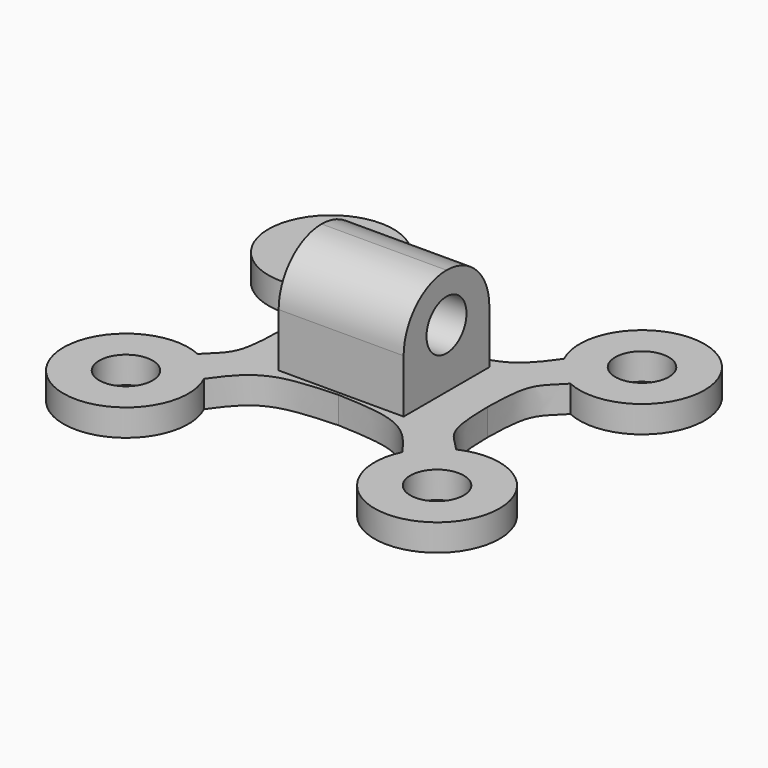
from build123d import *

# Parameters (mm, degrees)
F0_R     = 1.5
F0_W     = 7
F0_H     = 6
F1_DEPTH = 1.5
F2_DEPTH = 7.5
F3_R     = 1.4
F4_DEPTH = 25
F5_R     = 2.99999


# Not quite as in the source:
# - a fillet or chamfer is up to 0.001 mm smaller than in the source, because OpenCascade refuses the exact size


with BuildPart() as f1:
    # F0 (on Top) → F1 (new body)
    with BuildSketch(Plane.XY):
        with BuildLine():
            add(Edge.make_bspline(
                [(-5.5561550838, 5.6573497621), (-4.0955413133, 3.5522743128), (-3.2797986642, 3.3143495675), (0, 3.173440462)],
                knots=[0, 0, 0, 0, 6.0861042323, 6.0861042323, 6.0861042323, 6.0861042323], degree=3))
            ThreePointArc((-5.5561550838, 5.6573497621), (-11.1647533144, 9.6698318912), (-7.2436210565, 3.9969923231))
            add(Edge.make_bspline(
                [(-7.2436210565, 3.9969923231), (-6.2028751709, 2.9064782429), (-5.828993395, 2.9744568747), (-5.7950043119, 0)],
                knots=[0, 0, 0, 0, 4.2514042508, 4.2514042508, 4.2514042508, 4.2514042508], degree=3))
            add(Edge.make_bspline(
                [(-7.2436210565, -3.9969923231), (-6.2028751709, -2.9064782429), (-5.828993395, -2.9744568747), (-5.7950043119, 0)],
                knots=[0, 0, 0, 0, 4.2514042508, 4.2514042508, 4.2514042508, 4.2514042508], degree=3))
            ThreePointArc((-7.2436210565, -3.9969923231), (-11.1647533144, -9.6698318912), (-5.5561550838, -5.6573497621))
            add(Edge.make_bspline(
                [(-5.5561550838, -5.6573497621), (-4.0955413133, -3.5522743128), (-3.2797986642, -3.3143495675), (0, -3.173440462)],
                knots=[0, 0, 0, 0, 6.0861042323, 6.0861042323, 6.0861042323, 6.0861042323], degree=3))
            add(Edge.make_bspline(
                [(5.5561550838, -5.6573497621), (4.0955413133, -3.5522743128), (3.2797986642, -3.3143495675), (0, -3.173440462)],
                knots=[0, 0, 0, 0, 6.0861042323, 6.0861042323, 6.0861042323, 6.0861042323], degree=3))
            ThreePointArc((5.5561550838, -5.6573497621), (11.1647533144, -9.6698318912), (7.2436210565, -3.9969923231))
            add(Edge.make_bspline(
                [(7.2436210565, -3.9969923231), (6.2028751709, -2.9064782429), (5.828993395, -2.9744568747), (5.7950043119, 0)],
                knots=[0, 0, 0, 0, 4.2514042508, 4.2514042508, 4.2514042508, 4.2514042508], degree=3))
            add(Edge.make_bspline(
                [(7.2436210565, 3.9969923231), (6.2028751709, 2.9064782429), (5.828993395, 2.9744568747), (5.7950043119, 0)],
                knots=[0, 0, 0, 0, 4.2514042508, 4.2514042508, 4.2514042508, 4.2514042508], degree=3))
            ThreePointArc((7.2436210565, 3.9969923231), (11.1647533144, 9.6698318912), (5.5561550838, 5.6573497621))
            add(Edge.make_bspline(
                [(5.5561550838, 5.6573497621), (4.0955413133, 3.5522743128), (3.2797986642, 3.3143495675), (0, 3.173440462)],
                knots=[0, 0, 0, 0, 6.0861042323, 6.0861042323, 6.0861042323, 6.0861042323], degree=3))
        make_face()
        with Locations((-8.71, -7.175)):
            Circle(F0_R, mode=Mode.SUBTRACT)
        with Locations((8.71, -7.175)):
            Circle(F0_R, mode=Mode.SUBTRACT)
        with Locations((-8.71, 7.175)):
            Circle(F0_R, mode=Mode.SUBTRACT)
        Rectangle(F0_W, F0_H, mode=Mode.SUBTRACT)
        with Locations((8.71, 7.175)):
            Circle(F0_R, mode=Mode.SUBTRACT)
    extrude(amount=F1_DEPTH)

    # F0 (on Top) → F2 (join)
    with BuildSketch(Plane.XY):
        Rectangle(F0_W, F0_H)
    extrude(amount=F2_DEPTH)

    # F3 (on face) → F4 (cut)
    with BuildSketch(Plane(origin=(-3.5, 0, 0), x_dir=(0, -1, 0), z_dir=(-1, 0, 0))):
        with Locations((0, 4.8)):
            Circle(F3_R)
    extrude(amount=-F4_DEPTH, mode=Mode.SUBTRACT)

    # F5 (radius 3 in the source; OpenCascade refuses exactly that, so slightly less here)
    f5_edges = [f1.edges().sort_by_distance(p)[0] for p in [
        (0, 3, 7.5),
        (0, -3, 7.5),
    ]]
    fillet(f5_edges, radius=F5_R)


solid = f1.part
